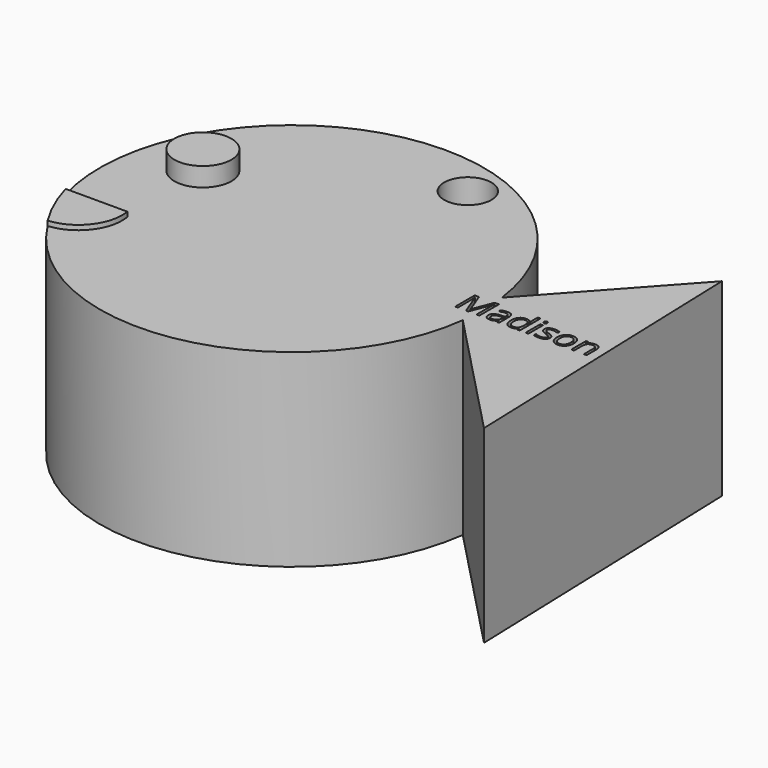
from build123d import *

# Parameters (mm, degrees)
F1_DEPTH     = 25.4
F2_R         = 3.8345875585
F3_DEPTH     = 2.54
F5_DEPTH     = 0.635
F6_TEXT_SIZE = 4.5964132167
F7_DEPTH     = 6.35
F8_R         = 3.175
F9_DEPTH     = 25.4


# Not quite as in the source:
# - Text() gives the source's letters only with a copy of the font that has no kerning and outlines rounded to 1/6400 em; it was checked with that copy


with BuildPart() as f1:
    # F0 (on Top) → F1 (new body)
    with BuildSketch(Plane.XY):
        with BuildLine():
            Line((71.0551068187, 62.8789067268), (55.3592814542, 45.5369946082))
            ThreePointArc((55.3592814542, 45.5369946082), (3.9990387156, 42.2310034183), (55.3625170355, 38.975668291))
            Line((55.3625170355, 38.975668291), (72.4178105593, 21.2191976607))
            Line((72.4178105593, 21.2191976607), (71.0551068187, 62.8789067268))
        make_face()
    extrude(amount=F1_DEPTH)

    # F2 (on face) → F3 (join)
    with BuildSketch(Plane.XY.offset(25.4)):
        with Locations((12.8483222798, 48.473212868)):
            Circle(F2_R)
    extrude(amount=F3_DEPTH)

    # F4 (on face) → F5 (join)
    with BuildSketch(Plane.XY.offset(25.4)):
        with BuildLine():
            Line((13.2376647532, 35.2977971467), (4.952166113, 35.2977971467))
            ThreePointArc((4.952166113, 35.2977971467), (6.2188892481, 31.7769505961), (7.9818418177, 28.4765042367))
            ThreePointArc((7.9818418177, 28.4765042367), (12.0991952349, 30.7395320126), (13.2376647532, 35.2977971467))
        make_face()
    extrude(amount=F5_DEPTH)

    # F6 (on face) → F7 (cut)
    with BuildSketch(Plane.XY.offset(25.4)):
        with Locations((52.3666441441, 40.8810265362)):
            Text('Madison', F6_TEXT_SIZE, font='Open Sans', text_align=(TextAlign.LEFT, TextAlign.BOTTOM))
    extrude(amount=-F7_DEPTH, mode=Mode.SUBTRACT)

    # F8 (on face) → F9 (cut)
    with BuildSketch(Plane.XY.offset(25.4)):
        with Locations((37.4642688258, 62.193105719)):
            Circle(F8_R)
    extrude(amount=-F9_DEPTH, mode=Mode.SUBTRACT)


solid = f1.part
